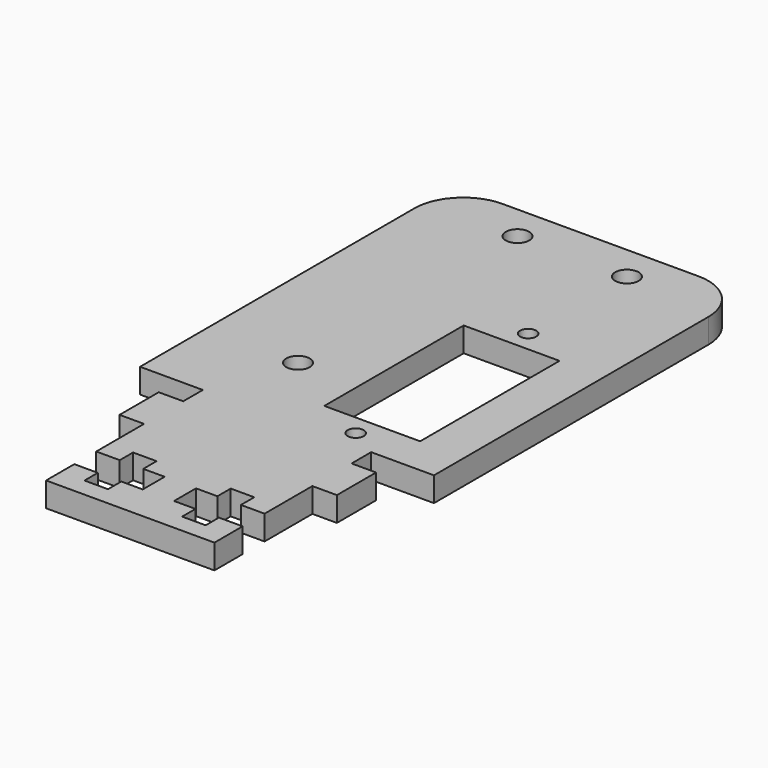
from build123d import *

# Parameters (mm, degrees)
F0_R     = 1.524
F0_R_2   = 1.04775
F0_W     = 12.4206
F0_H     = 22.5806
F1_DEPTH = 3.175


# Not quite as in the source:
# - ends of sketch curves that miss each other by under 0.0002 mm in the source are joined
# - a length typed as a fraction of an inch, garbled in the dataset ("3 / 203.2 mm" for 3/8 in), is restored


with BuildPart() as f1:
    # F0 (on Top) → F1 (new body)
    with BuildSketch(Plane.XY):
        with BuildLine():
            ThreePointArc((19.0496193061, 35.359281088), (17.1886928512, 39.8489739211), (12.6981263868, 41.7077912426))
            Line((12.6981263868, 41.7077912426), (-12.7018729111, 41.7018188664))
            ThreePointArc((-12.7018729111, 41.7018188664), (-17.19156232, 39.8408924124), (-19.0503796423, 35.3503293721))
            Line((-19.0503796423, 35.3503293721), (-19.0399523971, -9.0977780687))
            Line((-19.0399523971, -9.0977780687), (-10.8996863639, -9.0977780687))
            Line((-10.8996863639, -9.0977780687), (-10.8996863639, -12.2727780687))
            Line((-10.8996863639, -12.2727780687), (-14.0746863639, -12.2727780687))
            Line((-14.0746863639, -12.2727780687), (-14.0746863639, -18.6227780687))
            Line((-14.0746863639, -18.6227780687), (-10.8996939729, -18.6227780687))
            Line((-10.8996939729, -18.6227780687), (-10.8996939729, -26.3697780687))
            Line((-10.8996939729, -26.3697780687), (-7.8538059598, -26.3697780687))
            Line((-7.8538059598, -26.3697780687), (-7.8538059598, -24.2107780687))
            Line((-7.8538059598, -24.2107780687), (-4.8058059598, -24.2107780687))
            Line((-4.8058059598, -24.2107780687), (-4.8058059598, -26.3697780687))
            Line((-4.8058059598, -26.3697780687), (-2.0297826182, -26.3697780687))
            Line((-2.0297826182, -26.3697780687), (-2.0297826182, -29.9257780687))
            Line((-2.0297826182, -29.9257780687), (-4.8058059598, -29.9257780687))
            Line((-4.8058059598, -29.9257780687), (-4.8058059598, -32.0847780687))
            Line((-4.8058059598, -32.0847780687), (-7.8538059598, -32.0847780687))
            Line((-7.8538059598, -32.0847780687), (-7.8538059598, -29.9257780687))
            Line((-7.8538059598, -29.9257780687), (-10.8996939729, -29.9257780687))
            Line((-10.8996939729, -29.9257780687), (-10.8996939729, -34.4977780687))
            Line((-10.8996939729, -34.4977780687), (10.9197826182, -34.4977780687))
            Line((10.9197826182, -34.4977780687), (10.9197826182, -29.9257780687))
            Line((10.9197826182, -29.9257780687), (7.8538059598, -29.9257780687))
            Line((7.8538059598, -29.9257780687), (7.8538059598, -32.0847780687))
            Line((7.8538059598, -32.0847780687), (4.8058059598, -32.0847780687))
            Line((4.8058059598, -32.0847780687), (4.8058059598, -29.9257780687))
            Line((4.8058059598, -29.9257780687), (2.0297826182, -29.9257780687))
            Line((2.0297826182, -29.9257780687), (2.0297826182, -26.3697780687))
            Line((2.0297826182, -26.3697780687), (4.8058059598, -26.3697780687))
            Line((4.8058059598, -26.3697780687), (4.8058059598, -24.2107780687))
            Line((4.8058059598, -24.2107780687), (7.8538059598, -24.2107780687))
            Line((7.8538059598, -24.2107780687), (7.8538059598, -26.3697780687))
            Line((7.8538059598, -26.3697780687), (10.9197826182, -26.3697780687))
            Line((10.9197826182, -26.3697780687), (10.9197826182, -18.6227780687))
            Line((10.9197826182, -18.6227780687), (14.0947826182, -18.6227780687))
            Line((14.0947826182, -18.6227780687), (14.0947826182, -12.2727780687))
            Line((14.0947826182, -12.2727780687), (10.9197826182, -12.2727780687))
            Line((10.9197826182, -12.2727780687), (10.9197826182, -9.0977780687))
            Line((10.9197826182, -9.0977780687), (19.0600486513, -9.0977780687))
            Line((19.0600486513, -9.0977780687), (19.0496193061, 35.359281088))
        make_face()
        with Locations((-7.0950099938, 1.5702219313)):
            Circle(F0_R, mode=Mode.SUBTRACT)
        with Locations((7.0950099938, -6.8244780687)):
            Circle(F0_R_2, mode=Mode.SUBTRACT)
        with Locations((-7.0950099938, 37.1302219313)):
            Circle(F0_R, mode=Mode.SUBTRACT)
        with Locations((7.0950099938, 7.1455219313)):
            Rectangle(F0_W, F0_H, mode=Mode.SUBTRACT)
        with Locations((7.0950099938, 21.1155219313)):
            Circle(F0_R_2, mode=Mode.SUBTRACT)
        with Locations((7.0950099938, 37.1302219313)):
            Circle(F0_R, mode=Mode.SUBTRACT)
    extrude(amount=F1_DEPTH)


solid = f1.part
